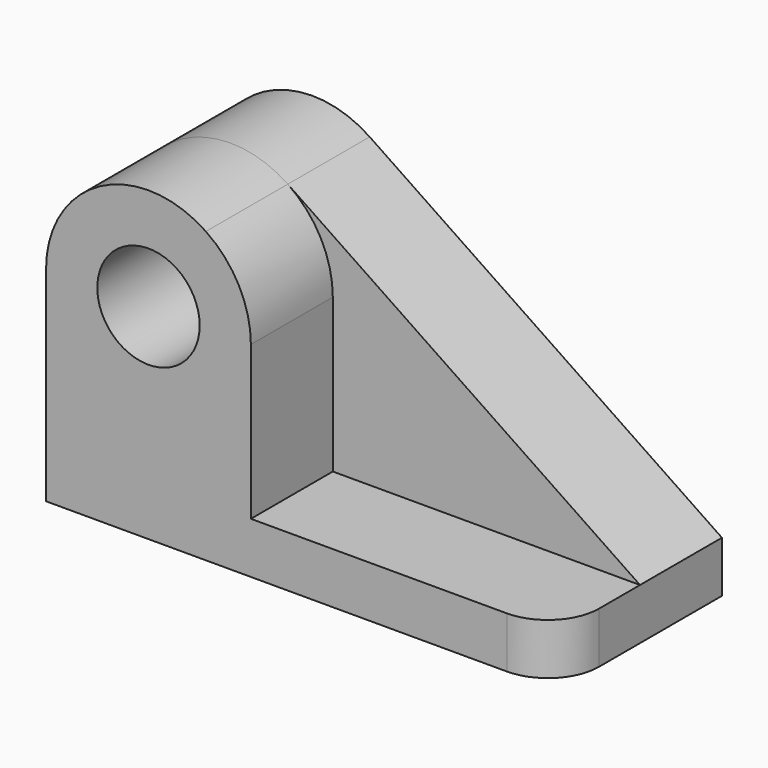
from build123d import *

# Parameters (mm, degrees)
F0_R     = 12.7
F1_DEPTH = 25.4
F2_R     = 12.7
F3_DEPTH = 25.4
F4_R     = 12.7


# Not quite as in the source:
# - ends of sketch curves that miss each other by under 0.0002 mm in the source are joined


with BuildPart() as f1:
    # F0 (on Front) → F1 (new body)
    with BuildSketch(Plane.XZ):
        with BuildLine():
            Line((63.2129007654, 12.7), (-24.1528646808, 71.8148155579))
            ThreePointArc((-24.1528646808, 71.8148155579), (-50.2855998854, 73.2187510696), (-63.7870992346, 50.8))
            ThreePointArc((-63.7870992346, 50.8), (-63.78710636, 50.7890156001), (-63.7871087352, 50.7780311981))
            Line((-63.7871087352, 50.7780311981), (-63.7870992346, 0))
            Line((-63.7870992346, 0), (63.2129007654, 0))
            Line((63.2129007654, 0), (63.2129007654, 12.7))
        make_face()
        with Locations((-38.3871087352, 50.7780311981)):
            Circle(F0_R, mode=Mode.SUBTRACT)
    extrude(amount=F1_DEPTH)

    # F2 (on face) → F3 (join)
    with BuildSketch(Plane.XZ.offset(25.4)):
        with BuildLine():
            Line((-12.9871182357, 12.7), (-12.9871182357, 50.7780311981))
            ThreePointArc((-12.9871182357, 50.7780311981), (-15.951544937, 62.6862214229), (-24.1528700049, 71.8148076894))
            ThreePointArc((-24.1528700049, 71.8148076894), (-50.2855954349, 73.2187426759), (-63.7870897341, 50.7999999918))
            ThreePointArc((-63.7870897341, 50.7999999918), (-63.7870968595, 50.789015596), (-63.7870992346, 50.7780311981))
            Line((-63.7870992346, 50.7780311981), (-63.7870992346, 12.7))
            Line((-63.7870992346, 12.7), (-63.7870992346, 0))
            Line((-63.7870992346, 0), (63.2129007654, 0))
            Line((63.2129007654, 0), (63.2129007654, 12.7))
            Line((63.2129007654, 12.7), (-12.9871182357, 12.7))
        make_face()
        with Locations((-38.3871087352, 50.7780311981)):
            Circle(F2_R, mode=Mode.SUBTRACT)
    extrude(amount=F3_DEPTH)

    # F4
    f4_edges = [f1.edges().sort_by_distance(p)[0] for p in [
        (63.212901, -50.8, 6.35),
    ]]
    fillet(f4_edges, radius=F4_R)


solid = f1.part
